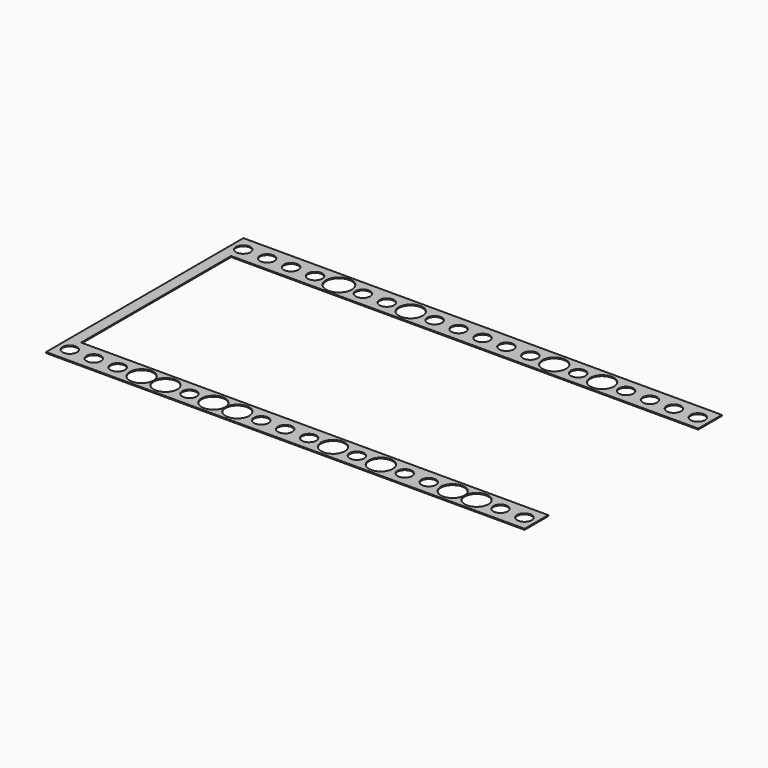
from build123d import *

# Parameters (mm, degrees)
F0_R     = 0.7326874882
F0_R_2   = 1.3
F0_R_3   = 1.2
F0_W     = 1.1555750221
F0_H     = 19
F1_DEPTH = 0.1


# Not quite as in the source:
# - a feature names something its author has since deleted; it is built from what else it names


with BuildPart() as f1:
    # F0 (on Top) → F1 (new body)
    with BuildSketch(Plane.XY):
        Polygon((24.25, 14.5), (-24.25, 14.5), (-24.25, 11.5), (-23.0944249779, 11.5), (-1.1800766224, 11.5), (1.0609005112, 11.5), (24.25, 11.5), align=None)
        with Locations((-23.0375, 12.9655366763)):
            Circle(F0_R, mode=Mode.SUBTRACT)
        with Locations((-20.6125, 12.9655366763)):
            Circle(F0_R, mode=Mode.SUBTRACT)
        with Locations((-18.1875, 12.9655366763)):
            Circle(F0_R, mode=Mode.SUBTRACT)
        with Locations((-15.7625, 12.9655366763)):
            Circle(F0_R, mode=Mode.SUBTRACT)
        with Locations((-13.3375, 12.9655366763)):
            Circle(F0_R_2, mode=Mode.SUBTRACT)
        with Locations((-10.9125, 12.9655366763)):
            Circle(F0_R, mode=Mode.SUBTRACT)
        with Locations((-8.4875, 12.9655366763)):
            Circle(F0_R, mode=Mode.SUBTRACT)
        with Locations((-6.0625, 12.9655366763)):
            Circle(F0_R_3, mode=Mode.SUBTRACT)
        with Locations((-3.6375, 12.9655366763)):
            Circle(F0_R, mode=Mode.SUBTRACT)
        with Locations((-1.2125, 12.9655366763)):
            Circle(F0_R, mode=Mode.SUBTRACT)
        with Locations((1.2125, 12.9655366763)):
            Circle(F0_R, mode=Mode.SUBTRACT)
        with Locations((3.6375, 12.9655366763)):
            Circle(F0_R, mode=Mode.SUBTRACT)
        with Locations((6.0625, 12.9655366763)):
            Circle(F0_R, mode=Mode.SUBTRACT)
        with Locations((8.4875, 12.9655366763)):
            Circle(F0_R_3, mode=Mode.SUBTRACT)
        with Locations((10.9125, 12.9655366763)):
            Circle(F0_R, mode=Mode.SUBTRACT)
        with Locations((13.3375, 12.9655366763)):
            Circle(F0_R_3, mode=Mode.SUBTRACT)
        with Locations((15.7625, 12.9655366763)):
            Circle(F0_R, mode=Mode.SUBTRACT)
        with Locations((18.1875, 12.9655366763)):
            Circle(F0_R, mode=Mode.SUBTRACT)
        with Locations((20.6125, 12.9655366763)):
            Circle(F0_R, mode=Mode.SUBTRACT)
        with Locations((23.0375, 12.9655366763)):
            Circle(F0_R, mode=Mode.SUBTRACT)
        Polygon((-23.0944249779, -7.5), (-24.25, -7.5), (-24.25, -10.5), (24.25, -10.5), (24.25, -7.5), (1.0609005112, -7.5), (-1.1800766224, -7.5), align=None)
        with Locations((-23.0375, -9.0053491294)):
            Circle(F0_R, mode=Mode.SUBTRACT)
        with Locations((-20.6125, -9.0053491294)):
            Circle(F0_R, mode=Mode.SUBTRACT)
        with Locations((-18.1875, -9.0053491294)):
            Circle(F0_R, mode=Mode.SUBTRACT)
        with Locations((-15.7625, -9.0053491294)):
            Circle(F0_R_3, mode=Mode.SUBTRACT)
        with Locations((-13.3375, -9.0053491294)):
            Circle(F0_R_3, mode=Mode.SUBTRACT)
        with Locations((-10.9125, -9.0053491294)):
            Circle(F0_R, mode=Mode.SUBTRACT)
        with Locations((-8.4875, -9.0053491294)):
            Circle(F0_R_3, mode=Mode.SUBTRACT)
        with Locations((-6.0625, -9.0053491294)):
            Circle(F0_R_3, mode=Mode.SUBTRACT)
        with Locations((-3.6375, -9.0053491294)):
            Circle(F0_R, mode=Mode.SUBTRACT)
        with Locations((-1.2125, -9.0053491294)):
            Circle(F0_R, mode=Mode.SUBTRACT)
        with Locations((1.2125, -9.0053491294)):
            Circle(F0_R, mode=Mode.SUBTRACT)
        with Locations((3.6375, -9.0053491294)):
            Circle(F0_R_3, mode=Mode.SUBTRACT)
        with Locations((6.0625, -9.0053491294)):
            Circle(F0_R, mode=Mode.SUBTRACT)
        with Locations((8.4875, -9.0053491294)):
            Circle(F0_R_3, mode=Mode.SUBTRACT)
        with Locations((10.9125, -9.0053491294)):
            Circle(F0_R, mode=Mode.SUBTRACT)
        with Locations((13.3375, -9.0053491294)):
            Circle(F0_R, mode=Mode.SUBTRACT)
        with Locations((15.7625, -9.0053491294)):
            Circle(F0_R_3, mode=Mode.SUBTRACT)
        with Locations((18.1875, -9.0053491294)):
            Circle(F0_R_3, mode=Mode.SUBTRACT)
        with Locations((20.6125, -9.0053491294)):
            Circle(F0_R, mode=Mode.SUBTRACT)
        with Locations((23.0375, -9.0053491294)):
            Circle(F0_R, mode=Mode.SUBTRACT)
        with Locations((-23.6722124889, 2)):
            Rectangle(F0_W, F0_H)
    extrude(amount=F1_DEPTH)


solid = f1.part
